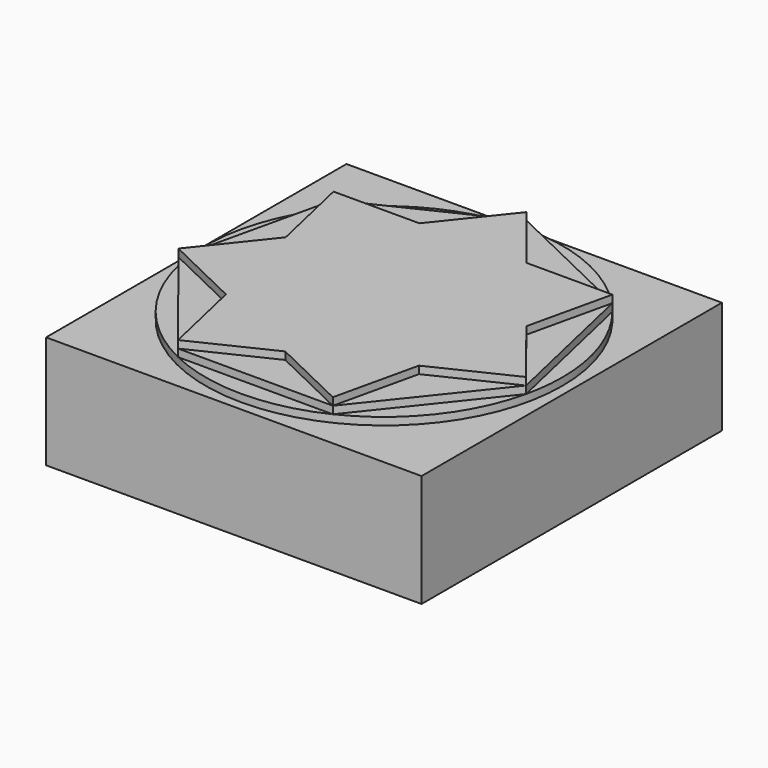
from build123d import *

# Parameters (mm, degrees)
F0_W     = 100
F0_H     = 100
F1_DEPTH = 30
F2_R     = 47.5
F3_DEPTH = 2
F5_DEPTH = 2
F7_DEPTH = 2


# Not quite as in the source:
# - a feature names something its author has since deleted; it is built from what else it names


with BuildPart() as f1:
    # F0 (on Top) → F1 (new body)
    with BuildSketch(Plane.XY):
        Rectangle(F0_W, F0_H)
    extrude(amount=F1_DEPTH)

    # F2 (on face) → F3 (join)
    with BuildSketch(Plane.XY.offset(30)):
        Circle(F2_R)
    extrude(amount=F3_DEPTH)

    # F4 (on face) → F5 (join)
    with BuildSketch(Plane.XY.offset(32)):
        Polygon((37.1369954172, 29.6157655883), (0, 47.5), (-37.1369954172, 29.6157655883), (-46.3090758286, -10.5697443629), (-20.6094776081, -42.7960212254), (20.6094776081, -42.7960212254), (46.3090758286, -10.5697443629), align=None)
    extrude(amount=F5_DEPTH)

    # F6 (on face) → F7 (join)
    with BuildSketch(Plane.XY.offset(34)):
        Polygon((-25.6995982206, -20.4947456859), (-20.6094776081, -42.7960212254), (0, -32.8710199024), (20.6094776081, -42.7960212254), (25.6995982206, -20.4947456859), (46.3090758286, -10.5697443629), (32.0468748048, 7.3144900488), (37.1369954172, 29.6157655883), (14.2622010239, 29.6157655883), (0, 47.5), (-14.2622010239, 29.6157655883), (-37.1369954172, 29.6157655883), (-32.0468748048, 7.3144900488), (-46.3090758286, -10.5697443629), align=None)
    extrude(amount=F7_DEPTH)


solid = f1.part
